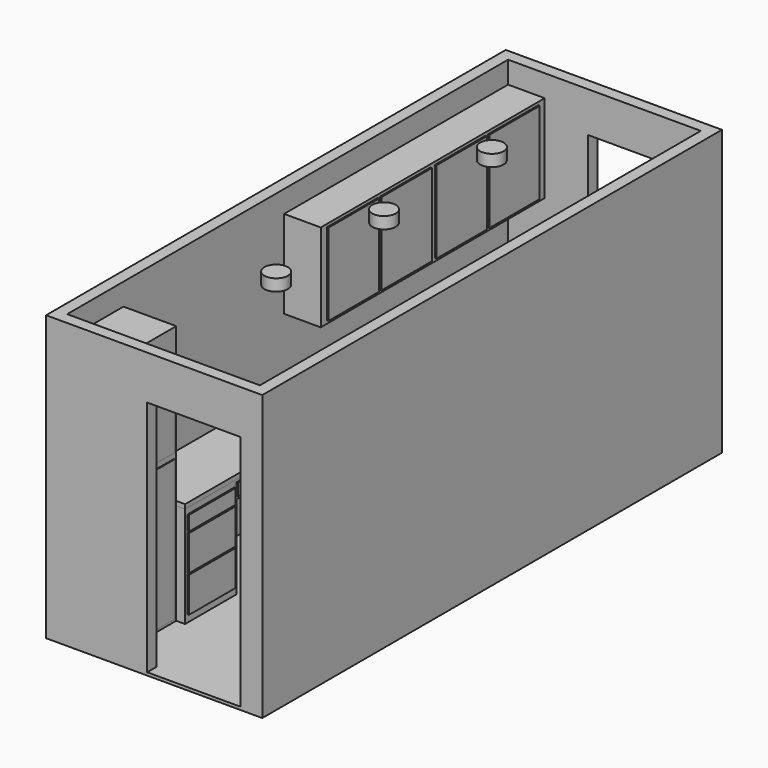
from build123d import *

# Parameters (mm, degrees)
F0_W      = 1873.25
F0_H      = 4978.4
F0_W_2    = 1670.05
F0_H_2    = 4775.2
F1_DEPTH  = 2438.4
F2_W      = 806.45
F2_H      = 2057.4
F3_DEPTH  = 101.6
F4_W      = 895.35
F4_H      = 914.4
F5_DEPTH  = 101.6
F6_W      = 1873.25
F6_H      = 4978.4
F6_W_2    = 254
F6_H_2    = 101.6
F7_DEPTH  = 25.4
F8_W      = 635
F8_H      = 685.8
F9_DEPTH  = 914.4
F10_W     = 2425.7
F10_H     = 762
F11_DEPTH = 317.5
F13_W     = 76.2
F13_H     = 114.3
F14_DEPTH = 6.35
F15_R     = 101.6
F16_DEPTH = 101.6
F17_W     = 609.6
F17_H     = 2247.9
F18_DEPTH = 457.2
F19_W     = 914.4
F19_H     = 914.4
F20_DEPTH = 609.6
F21_W     = 1727.2
F21_H     = 38.1
F22_DEPTH = 533.4
F23_W     = 1168.4
F23_H     = 152.4
F24_DEPTH = 533.4
F25_W     = 508
F25_H     = 304.8
F25_H_2   = 127
F25_W_2   = 1134.1810718536
F25_H_3   = 104.1873693466
F26_DEPTH = 12.7
F12_R     = 19.05
F27_DEPTH = 101.6
F28_W     = 266.7
F28_H     = 1219.2
F28_H_2   = 609.6
F29_DEPTH = 6.35
F30_W     = 546.1
F30_H     = 711.2
F31_DEPTH = 12.7
F32_W     = 76.2
F32_H     = 127
F33_DEPTH = 6.35
F34_W     = 76.2
F34_H     = 127
F35_DEPTH = 6.35
F36_W     = 381
F36_H     = 635
F37_DEPTH = 304.8


# Not quite as in the source:
# - a feature names something its author has since deleted; it is built from what else it names


with BuildPart() as f1:
    # F0 (on Top) → F1 (new body)
    with BuildSketch(Plane.XY):
        with Locations((-835.025, 2387.6)):
            Rectangle(F0_W, F0_H)
        with Locations((-835.025, 2387.6)):
            Rectangle(F0_W_2, F0_H_2, mode=Mode.SUBTRACT)
    extrude(amount=F1_DEPTH)

    # F2 (on face) → F3 (cut, through all)
    with BuildSketch(Plane.XZ.offset(101.6)):
        with Locations((-492.125, 1028.7)):
            Rectangle(F2_W, F2_H)
    extrude(amount=-F3_DEPTH, mode=Mode.SUBTRACT)

    # F4 (on face) → F5 (cut, through all)
    with BuildSketch(Plane.XZ.offset(-4775.2)):
        with Locations((-530.225, 1631.95)):
            Rectangle(F4_W, F4_H)
    extrude(amount=-F5_DEPTH, mode=Mode.SUBTRACT)

    # F6 (on face) → F7 (join)
    with BuildSketch(Plane(origin=(0, 0, 0), x_dir=(1, 0, 0), z_dir=(0, 0, -1))):
        with Locations((-835.025, -2387.6)):
            Rectangle(F6_W, F6_H)
        with Locations((-1060.45, -2489.2)):
            Rectangle(F6_W_2, F6_H_2, mode=Mode.SUBTRACT)
    extrude(amount=F7_DEPTH)

    # F12 (on face) → F27 (cut, through all)
    with BuildSketch(Plane(origin=(-1771.65, 0, 0), x_dir=(0, -1, 0), z_dir=(-1, 0, 0))):
        with Locations((-2743.2, 431.8)):
            Circle(F12_R)
    extrude(amount=-F27_DEPTH, mode=Mode.SUBTRACT)


with BuildPart() as f9:
    # F8 (on face) → F9 (new body)
    with BuildSketch(Plane.XY):
        with Locations((-1225.55, 4381.5)):
            Rectangle(F8_W, F8_H)
    extrude(amount=F9_DEPTH)


with BuildPart() as f9b:
    # F8 (on face) → F9, piece 2 (new body)
    with BuildSketch(Plane.XY):
        with Locations((-1225.55, 3670.3)):
            Rectangle(F8_W, F8_H)
    extrude(amount=F9_DEPTH)


with BuildPart() as f11:
    # F10 (on face) → F11 (new body)
    with BuildSketch(Plane.YZ.offset(-1670.05)):
        with Locations((3562.35, 1866.9)):
            Rectangle(F10_W, F10_H)
    extrude(amount=F11_DEPTH)

    # F30 (on face) → F31 (join)
    with BuildSketch(Plane.YZ.offset(-1352.55)):
        with Locations((2692.4, 1866.9)):
            Rectangle(F30_W, F30_H)
        with Locations((3263.9, 1866.9)):
            Rectangle(F30_W, F30_H)
        with Locations((3860.8, 1866.9)):
            Rectangle(F30_W, F30_H)
        with Locations((4432.3, 1866.9)):
            Rectangle(F30_W, F30_H)
    extrude(amount=F31_DEPTH)


with BuildPart() as f14:
    # F13 (on face) → F14 (new body)
    with BuildSketch(Plane(origin=(0, 0, 0), x_dir=(-1, 0, 0), z_dir=(0, 1, 0))):
        with Locations((1047.75, 1225.55)):
            Rectangle(F13_W, F13_H)
    extrude(amount=F14_DEPTH)


with BuildPart() as f16:
    # F15 (on face) → F16 (new body)
    with BuildSketch(Plane.XY.offset(2438.4)):
        with Locations((-835.025, 3556)):
            Circle(F15_R)
    extrude(amount=F16_DEPTH)


with BuildPart() as f16b:
    # F15 (on face) → F16, piece 2 (new body)
    with BuildSketch(Plane.XY.offset(2438.4)):
        with Locations((-835.025, 1219.2)):
            Circle(F15_R)
    extrude(amount=F16_DEPTH)


with BuildPart() as f16c:
    # F15 (on face) → F16, piece 3 (new body)
    with BuildSketch(Plane.XY.offset(2438.4)):
        with Locations((-835.025, 2387.6)):
            Circle(F15_R)
    extrude(amount=F16_DEPTH)


with BuildPart() as f18:
    # F17 (on face) → F18 (new body)
    with BuildSketch(Plane.YZ.offset(-1670.05)):
        with Locations((304.8, 1123.95)):
            Rectangle(F17_W, F17_H)
    extrude(amount=F18_DEPTH)

    # F28 (on face) → F29 (join)
    with BuildSketch(Plane.YZ.offset(-1212.85)):
        with Locations((158.75, 635)):
            Rectangle(F28_W, F28_H)
        with Locations((450.85, 635)):
            Rectangle(F28_W, F28_H)
        with Locations((158.75, 1600.2)):
            Rectangle(F28_W, F28_H_2)
        with Locations((450.85, 1600.2)):
            Rectangle(F28_W, F28_H_2)
    extrude(amount=F29_DEPTH)


with BuildPart() as f20:
    # F19 (on face) → F20 (new body)
    with BuildSketch(Plane.YZ.offset(-1670.05)):
        with Locations((2794, 457.2)):
            Rectangle(F19_W, F19_H)
    extrude(amount=F20_DEPTH)

    # F36 (on face) → F37 (cut)
    with BuildSketch(Plane.XY.offset(914.4)):
        with Locations((-1365.25, 2794)):
            Rectangle(F36_W, F36_H)
    extrude(amount=-F37_DEPTH, mode=Mode.SUBTRACT)


with BuildPart() as f22:
    # F21 (on face) → F22 (new body)
    with BuildSketch(Plane.YZ.offset(-1670.05)):
        with Locations((1473.2, 895.35)):
            Rectangle(F21_W, F21_H)
    extrude(amount=F22_DEPTH)


with BuildPart() as f24:
    # F23 (on face) → F24 (new body, through all)
    with BuildSketch(Plane.YZ.offset(-1136.65)):
        Polygon((1168.4, 876.3), (609.6, 876.3), (609.6, 0), (1168.4, 0), (1168.4, 723.9), align=None)
        with Locations((1752.6, 800.1)):
            Rectangle(F23_W, F23_H)
    extrude(amount=-F24_DEPTH)

    # F25 (on face) → F26 (join)
    with BuildSketch(Plane.YZ.offset(-1136.65)):
        with Locations((889, 215.9)):
            Rectangle(F25_W, F25_H)
        with Locations((889, 533.4)):
            Rectangle(F25_W, F25_H)
        with Locations((889, 762)):
            Rectangle(F25_W, F25_H_2)
        with Locations((1735.4905359268, 803.0257225037)):
            Rectangle(F25_W_2, F25_H_3)
    extrude(amount=F26_DEPTH)


with BuildPart() as f33:
    # F32 (on face) → F33 (new body)
    with BuildSketch(Plane(origin=(-1771.65, 0, 0), x_dir=(0, -1, 0), z_dir=(-1, 0, 0))):
        with Locations((-698.5, 292.1)):
            Rectangle(F32_W, F32_H)
    extrude(amount=F33_DEPTH)


with BuildPart() as f33b:
    # F32 (on face) → F33, piece 2 (new body)
    with BuildSketch(Plane(origin=(-1771.65, 0, 0), x_dir=(0, -1, 0), z_dir=(-1, 0, 0))):
        with Locations((-2882.9, 292.1)):
            Rectangle(F32_W, F32_H)
    extrude(amount=F33_DEPTH)


with BuildPart() as f35:
    # F34 (on face) → F35 (new body)
    with BuildSketch(Plane.YZ.offset(-1670.05)):
        with Locations((698.5, 1117.6)):
            Rectangle(F34_W, F34_H)
    extrude(amount=F35_DEPTH)


solid = Compound([f1.part, f9.part, f9b.part, f11.part, f14.part, f16.part, f16b.part, f16c.part, f18.part, f20.part, f22.part, f24.part, f33.part, f33b.part, f35.part])
